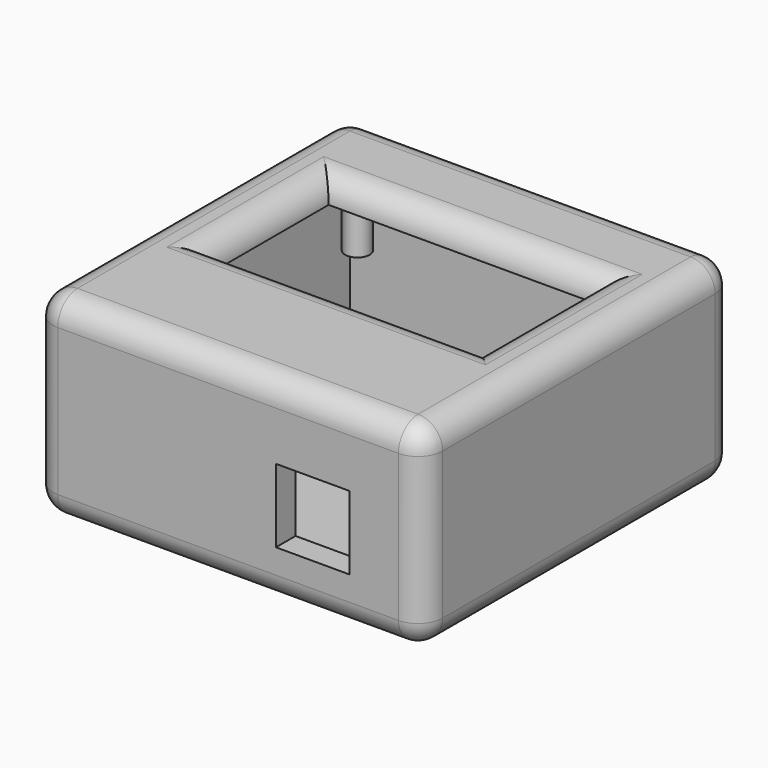
from build123d import *

# Parameters (mm, degrees)
F0_W      = 27.8
F0_H      = 27.8
F0_R      = 1
F0_W_2    = 22
F0_H_2    = 12
F1_DEPTH  = 2
F2_R      = 1.99999
F3_DEPTH  = 12
F4_W      = 27.8
F4_H      = 27.8
F5_DEPTH  = 2
F7_W      = 6
F7_H      = 6
F8_DEPTH  = 5
F9_R      = 2
F10_DEPTH = 5
F11_DEPTH = 5
F12_R     = 1.99999
F13_W     = 15.5
F13_H     = 15.5
F14_DEPTH = 1


# Not quite as in the source:
# - a fillet or chamfer is up to 0.001 mm smaller than in the source, because OpenCascade refuses the exact size
# - a feature names something its author has since deleted; it is built from what else it names


with BuildPart() as f1:
    # F0 (on Top) → F1 (new body)
    with BuildSketch(Plane.XY):
        with BuildLine():
            ThreePointArc((13.9, -15.9), (15.3142135624, -15.3142135624), (15.9, -13.9))
            Line((15.9, -13.9), (15.9, 13.9))
            ThreePointArc((15.9, 13.9), (15.3142135624, 15.3142135624), (13.9, 15.9))
            Line((13.9, 15.9), (-13.9, 15.9))
            ThreePointArc((-13.9, 15.9), (-15.3142135624, 15.3142135624), (-15.9, 13.9))
            Line((-15.9, 13.9), (-15.9, -13.9))
            ThreePointArc((-15.9, -13.9), (-15.3142135624, -15.3142135624), (-13.9, -15.9))
            Line((-13.9, -15.9), (13.9, -15.9))
        make_face()
        Rectangle(F0_W, F0_H, mode=Mode.SUBTRACT)
        Rectangle(F0_W, F0_H)
        with Locations((-11.65, -11.85)):
            Circle(F0_R, mode=Mode.SUBTRACT)
        with Locations((11.65, -11.85)):
            Circle(F0_R, mode=Mode.SUBTRACT)
        with Locations((0, 2.1)):
            Rectangle(F0_W_2, F0_H_2, mode=Mode.SUBTRACT)
        with Locations((-11.65, 11.85)):
            Circle(F0_R, mode=Mode.SUBTRACT)
        with Locations((11.65, 11.85)):
            Circle(F0_R, mode=Mode.SUBTRACT)
        with Locations((-11.65, -11.85)):
            Circle(F0_R)
        with Locations((11.65, -11.85)):
            Circle(F0_R)
        with Locations((11.65, 11.85)):
            Circle(F0_R)
        with Locations((-11.65, 11.85)):
            Circle(F0_R)
    extrude(amount=F1_DEPTH)

    # F2 (radius 2 in the source; OpenCascade refuses exactly that, so slightly less here)
    f2_edges = [f1.edges().sort_by_distance(p)[0] for p in [
        (0, 8.1, 2),
        (-11, 2.1, 2),
        (11, 2.1, 2),
        (0, -3.9, 2),
        (-15.9, 0, 2),
    ]]
    fillet(f2_edges, radius=F2_R)

    # F0 (on Top) → F3 (join)
    with BuildSketch(Plane.XY):
        with BuildLine():
            ThreePointArc((13.9, -15.9), (15.3142135624, -15.3142135624), (15.9, -13.9))
            Line((15.9, -13.9), (15.9, 13.9))
            ThreePointArc((15.9, 13.9), (15.3142135624, 15.3142135624), (13.9, 15.9))
            Line((13.9, 15.9), (-13.9, 15.9))
            ThreePointArc((-13.9, 15.9), (-15.3142135624, 15.3142135624), (-15.9, 13.9))
            Line((-15.9, 13.9), (-15.9, -13.9))
            ThreePointArc((-15.9, -13.9), (-15.3142135624, -15.3142135624), (-13.9, -15.9))
            Line((-13.9, -15.9), (13.9, -15.9))
        make_face()
        Rectangle(F0_W, F0_H, mode=Mode.SUBTRACT)
    extrude(amount=-F3_DEPTH)


with BuildPart() as f5:
    # F4 (on face) → F5 (new body)
    with BuildSketch(Plane(origin=(0, 0, -12), x_dir=(1, 0, 0), z_dir=(0, 0, -1))):
        with BuildLine():
            ThreePointArc((-13.9, 15.9), (-15.3142135624, 15.3142135624), (-15.9, 13.9))
            Line((-15.9, 13.9), (-15.9, -13.9))
            ThreePointArc((-15.9, -13.9), (-15.3142135624, -15.3142135624), (-13.9, -15.9))
            Line((-13.9, -15.9), (13.9, -15.9))
            ThreePointArc((13.9, -15.9), (15.3142135624, -15.3142135624), (15.9, -13.9))
            Line((15.9, -13.9), (15.9, 13.9))
            ThreePointArc((15.9, 13.9), (15.3142135624, 15.3142135624), (13.9, 15.9))
            Line((13.9, 15.9), (-13.9, 15.9))
        make_face()
        Rectangle(F4_W, F4_H, mode=Mode.SUBTRACT)
        Rectangle(F4_W, F4_H)
    extrude(amount=F5_DEPTH)

    # F6: cut F1
    add(f1.part, mode=Mode.SUBTRACT)

    # F12 (radius 2 in the source; OpenCascade refuses exactly that, so slightly less here)
    f12_edges = [f5.edges().sort_by_distance(p)[0] for p in [
        (0, -15.9, -14),
    ]]
    fillet(f12_edges, radius=F12_R)

    # F13 (on face) → F14 (cut)
    with BuildSketch(Plane(origin=(0, 0, -14), x_dir=(1, 0, 0), z_dir=(0, 0, -1))):
        with Locations((0, -6.15)):
            Rectangle(F13_W, F13_H)
    extrude(amount=-F14_DEPTH, mode=Mode.SUBTRACT)


with BuildPart() as f1_1:
    add(f1.part)

    # F7 (on face) → F8 (cut)
    with BuildSketch(Plane.XZ.offset(15.9)):
        with Locations((6.9, -7)):
            Rectangle(F7_W, F7_H)
    extrude(amount=-F8_DEPTH, mode=Mode.SUBTRACT)

    # F9 (on face) → F10 (cut)
    with BuildSketch(Plane(origin=(-15.9, 0, 0), x_dir=(0, -1, 0), z_dir=(-1, 0, 0))):
        with Locations((7.9, -7)):
            Circle(F9_R)
    extrude(amount=-F10_DEPTH, mode=Mode.SUBTRACT)

    # F0 (on Top) → F11 (join)
    with BuildSketch(Plane.XY):
        with Locations((-11.65, -11.85)):
            Circle(F0_R)
        with Locations((11.65, -11.85)):
            Circle(F0_R)
        with Locations((-11.65, 11.85)):
            Circle(F0_R)
        with Locations((11.65, 11.85)):
            Circle(F0_R)
    extrude(amount=-F11_DEPTH)


solid = Compound([f5.part, f1_1.part])
